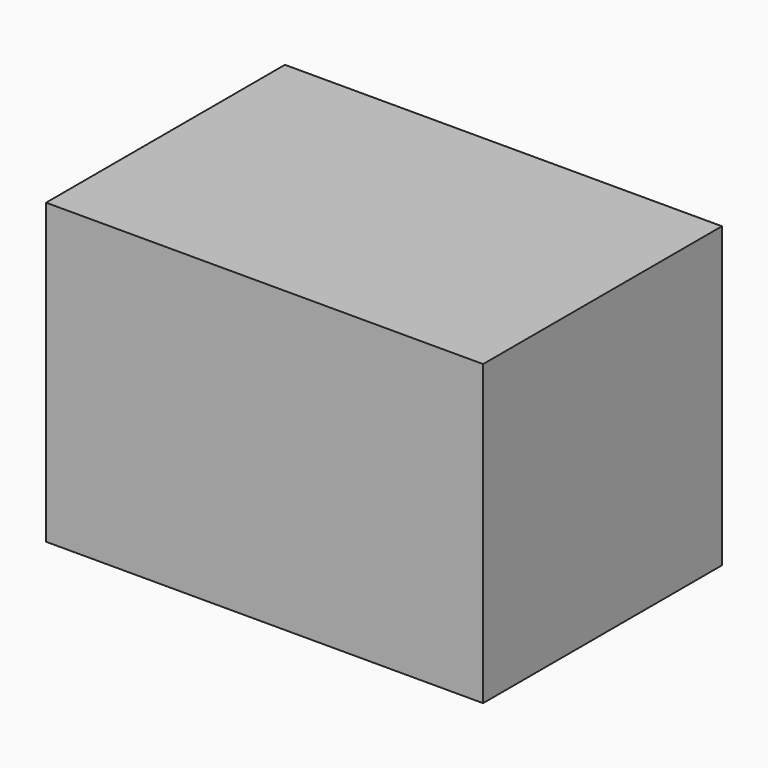
from build123d import *

# Parameters (mm, degrees)
F1_E0_TOP_W = 74.3621811271
F1_E0_TOP_H = 50.8
F2_DEPTH    = 50.8
F3_R        = 17.9542395823
F4_DEPTH    = 50.8


with BuildPart() as f2:
    # F1_E0_top (on explicit) → F2 (new body)
    with BuildSketch(Plane(origin=(-35.5028994381, -30.8898929507, 0), x_dir=(1, 0, 0), z_dir=(0, -1, 0))):
        with Locations((37.1810905635, 25.4)):
            Rectangle(F1_E0_TOP_W, F1_E0_TOP_H)
    extrude(amount=F2_DEPTH)

    # F3 (on face) → F4 (join)
    with BuildSketch(Plane.XY.offset(50.8)):
        with Locations((0, -52.5342226028)):
            Circle(F3_R)
    extrude(amount=-F4_DEPTH)


solid = f2.part
